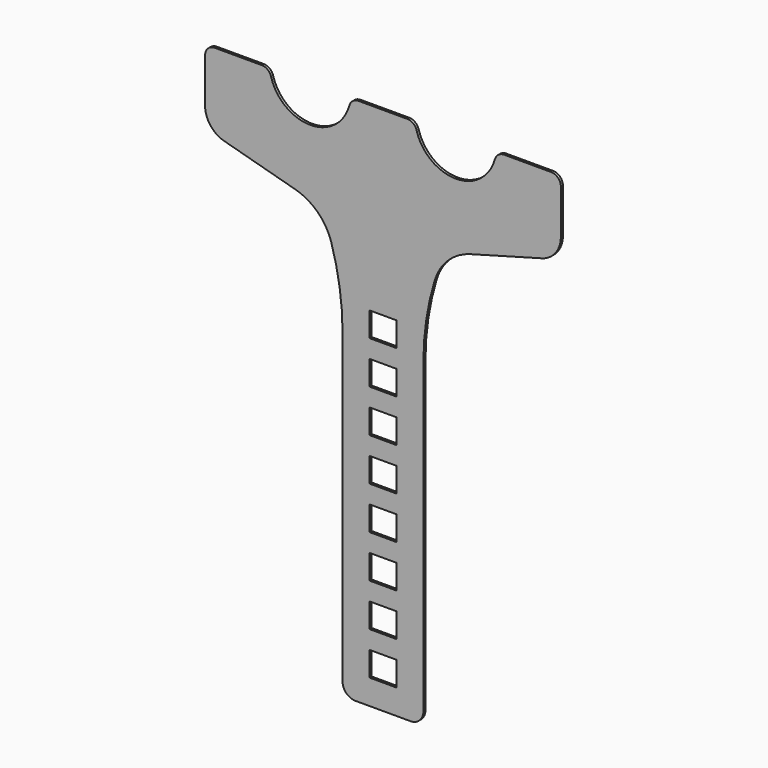
from build123d import *

# Parameters (mm, degrees)
F0_W        = 10.4902
F0_H        = 9.6012
F1_DEPTH    = 1.00584
F2_R        = 20.32
F3_R        = 10.16
F4_R        = 3.81
F5_R        = 3.81
F6_T1_DEPTH = 1.00584
F7_R        = 5.08


# Not quite as in the source:
# - a fillet or chamfer that OpenCascade refuses, or shapes differently, is made with other operations: its cross-section is extruded or revolved along the edge and cut away or added


with BuildPart() as f1:
    # F0 (on Front) → F1 (new body)
    with BuildSketch(Plane.XZ):
        with BuildLine():
            Line((-44.45, 0), (-69.85, 0))
            Line((-69.85, 0), (-69.85, -28.956))
            Line((-69.85, -28.956), (-23.7198378891, -41.5853487635))
            Line((-23.7198378891, -41.5853487635), (-15.875, -66.2231149459))
            Line((-15.875, -66.2231149459), (-15.875, -207.772))
            Line((-15.875, -207.772), (0, -207.772))
            Line((0, -207.772), (15.875, -207.772))
            Line((15.875, -207.772), (15.875, -66.2231149459))
            Line((15.875, -66.2231149459), (23.7198378891, -41.5853487635))
            Line((23.7198378891, -41.5853487635), (69.85, -28.956))
            Line((69.85, -28.956), (69.85, 0))
            Line((69.85, 0), (44.45, 0))
            ThreePointArc((44.45, 0), (28.575, -14.478), (12.7, 0))
            Line((12.7, 0), (-12.7, 0))
            ThreePointArc((-12.7, 0), (-28.575, -14.478), (-44.45, 0))
        make_face()
        with Locations((0, -193.1416)):
            Rectangle(F0_W, F0_H, mode=Mode.SUBTRACT)
        with Locations((0, -176.3776)):
            Rectangle(F0_W, F0_H, mode=Mode.SUBTRACT)
        with Locations((0, -159.6136)):
            Rectangle(F0_W, F0_H, mode=Mode.SUBTRACT)
        with Locations((0, -142.8496)):
            Rectangle(F0_W, F0_H, mode=Mode.SUBTRACT)
        with Locations((0, -126.0856)):
            Rectangle(F0_W, F0_H, mode=Mode.SUBTRACT)
        with Locations((0, -109.3216)):
            Rectangle(F0_W, F0_H, mode=Mode.SUBTRACT)
        with Locations((0, -92.5576)):
            Rectangle(F0_W, F0_H, mode=Mode.SUBTRACT)
        with Locations((0, -75.7936)):
            Rectangle(F0_W, F0_H, mode=Mode.SUBTRACT)
    extrude(amount=-F1_DEPTH)

    # F2
    f2_edges = [f1.edges().sort_by_distance(p)[0] for p in [
        (-23.719838, 0.50292, -41.585349),
        (23.719838, 0.50292, -41.585349),
    ]]
    fillet(f2_edges, radius=F2_R)

    # F3
    f3_edges = [f1.edges().sort_by_distance(p)[0] for p in [
        (-69.85, 0.50292, -28.956),
        (69.85, 0.50292, -28.956),
    ]]
    fillet(f3_edges, radius=F3_R)

    # F4
    f4_edges = [f1.edges().sort_by_distance(p)[0] for p in [
        (69.85, 0.50292, 0),
        (-69.85, 0.50292, 0),
    ]]
    fillet(f4_edges, radius=F4_R)

    # F5
    f5_edges = [f1.edges().sort_by_distance(p)[0] for p in [
        (44.45, 0.50292, 0),
        (-44.45, 0.50292, 0),
        (-12.7, 0.50292, 0),
        (12.7, 0.50292, 0),
    ]]
    fillet(f5_edges, radius=F5_R)

    # F6: fillet of radius 101.6 on 2 edges, made by hand

    # F6_s2 → F6_t1 (join)
    with BuildSketch(Plane.XZ.offset(-1.00584)):
        with BuildLine():
            ThreePointArc((15.875, -81.9921288589), (17.0051850195, -66.880005322), (20.3705960196, -52.1040923291))
            Line((20.3705960196, -52.1040923291), (18.42850794, -51.5063315985))
            ThreePointArc((18.42850794, -51.5063315985), (16.1865788547, -58.5470978522), (13.9387808449, -65.6066091605))
            Line((13.9387808449, -65.6066091605), (13.843, -66.2231149459))
            Line((13.843, -66.2231149459), (13.843, -81.9921288589))
            Line((13.843, -81.9921288589), (15.875, -81.9921288589))
        make_face()
        with BuildLine():
            ThreePointArc((-20.3705960196, -52.1040923291), (-17.0051850195, -66.880005322), (-15.875, -81.9921288589))
            Line((-15.875, -81.9921288589), (-13.843, -81.9921288589))
            Line((-13.843, -81.9921288589), (-13.843, -66.2231149459))
            Line((-13.843, -66.2231149459), (-13.9387808449, -65.6066091605))
            ThreePointArc((-13.9387808449, -65.6066091605), (-16.1865788547, -58.5470978522), (-18.42850794, -51.5063315985))
            Line((-18.42850794, -51.5063315985), (-20.3705960196, -52.1040923291))
        make_face()
    extrude(amount=F6_T1_DEPTH)

    # F7
    f7_edges = [f1.edges().sort_by_distance(p)[0] for p in [
        (15.875, 0.50292, -207.772),
        (-15.875, 0.50292, -207.772),
    ]]
    fillet(f7_edges, radius=F7_R)


solid = f1.part
